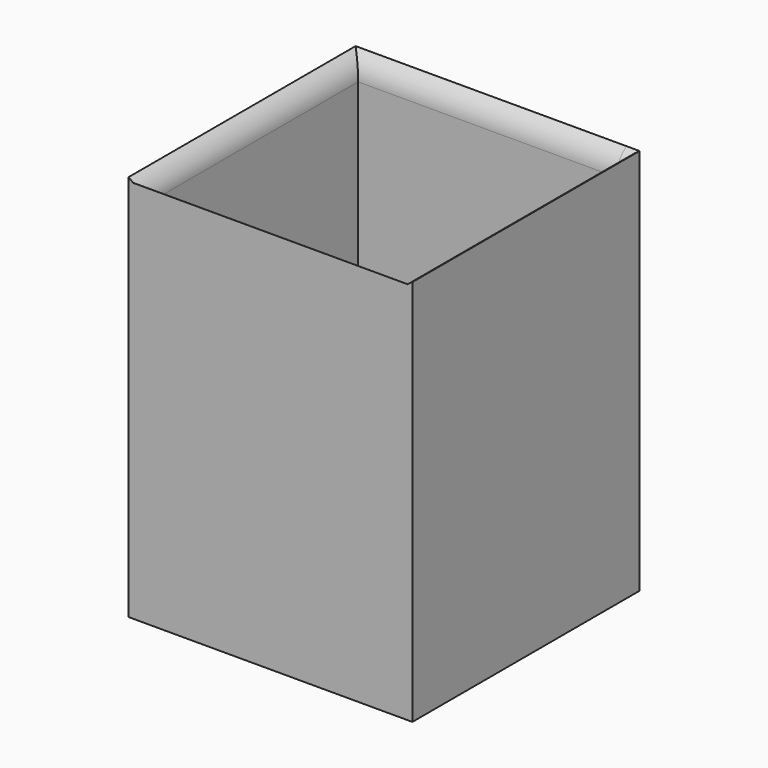
from build123d import *

# Parameters (mm, degrees)
F0_W         = 50.8
F0_H         = 50.8
F0_R         = 1.5875
F1_DEPTH     = 5.08
F0_W_2       = 55.88
F0_H_2       = 55.88
F2_DEPTH     = 76.2
F3_T1_DEPTH  = 50.8
F4_T4_DEPTH  = 64.3399164321
F4_S5_R      = 5.0800000001
F4_T6_DEPTH  = 34
F5_T4_DEPTH  = 64.3391166785
F5_S5_R      = 5.0813656856
F5_T6_DEPTH  = 34
F6_T4_DEPTH  = 77.8762455026
F6_S6_R      = 5.0800000001
F6_T7_DEPTH  = 41
F6_T11_DEPTH = 77.8762455026
F6_S13_R     = 5.081365685
F6_T14_DEPTH = 41
F7_R         = 5.7567075364
F8_DEPTH     = 8.128
F9_R         = 5.08


# Not quite as in the source:
# - a fillet or chamfer that OpenCascade refuses, or shapes differently, is made with other operations: its cross-section is extruded or revolved along the edge and cut away or added


with BuildPart() as f1:
    # F0 (on Top) → F1 (new body)
    with BuildSketch(Plane.XY):
        with Locations((0.627800245, -0.8074334759)):
            Rectangle(F0_W, F0_H)
        with Locations((-12.072199755, -13.5074334759)):
            Circle(F0_R, mode=Mode.SUBTRACT)
        with Locations((13.327800245, -13.5074334759)):
            Circle(F0_R, mode=Mode.SUBTRACT)
        with Locations((-12.072199755, 11.8925665241)):
            Circle(F0_R, mode=Mode.SUBTRACT)
        with Locations((13.327800245, 11.8925665241)):
            Circle(F0_R, mode=Mode.SUBTRACT)
    extrude(amount=F1_DEPTH)

    # F0 (on Top) → F2 (join)
    with BuildSketch(Plane.XY):
        with Locations((0.627800245, -0.8074334759)):
            Rectangle(F0_W_2, F0_H_2)
        with Locations((0.627800245, -0.8074334759)):
            Rectangle(F0_W, F0_H, mode=Mode.SUBTRACT)
    extrude(amount=F2_DEPTH)

    # F3: fillet of radius 5.08 on 1 edges, made by hand

    # F3_s2 → F3_t1 (cut)
    with BuildSketch(Plane.YZ.offset(-24.772199755)):
        with BuildLine():
            ThreePointArc((-26.2074334759, 71.12), (-27.6953310275, 74.7121024484), (-31.2874334759, 76.2))
            Line((-31.2874334759, 76.2), (-26.2074334759, 76.2))
            Line((-26.2074334759, 76.2), (-26.2074334759, 71.12))
        make_face()
    extrude(amount=F3_T1_DEPTH, mode=Mode.SUBTRACT)

    # F4: fillet of radius 5.08 on 1 edges, made by hand


with BuildPart() as f4_tool2:
    # F4_s3 → F4_t4 (new body)
    with BuildSketch(Plane.XZ.offset(-24.5925665241)):
        with BuildLine():
            ThreePointArc((-27.311999717, 76.2003463882), (-25.4524342775, 74.3404748362), (-24.771799755, 71.8000334454))
            Line((-24.771799755, 71.8000334454), (-24.2636631865, 71.8000334454))
            ThreePointArc((-24.2636631865, 71.8000334454), (-24.2640631865, 74.0000167227), (-24.2640631865, 76.2))
            Line((-24.2640631865, 76.2), (-24.772199755, 76.7081365685))
            ThreePointArc((-24.772199755, 76.7081365685), (-26.042099736, 76.7081365685), (-27.0578831447, 76.6403776825))
            Line((-27.0578831447, 76.6403776825), (-27.311999717, 76.2003463882))
        make_face()
    extrude(amount=F4_T4_DEPTH)

    # F4_s5 → F4_t6 (cut, symmetric)
    with BuildSketch(Plane.YZ.offset(-25.8)):
        with Locations((-31.287433476, 71.1199999999)):
            Circle(F4_S5_R)
    extrude(amount=F4_T6_DEPTH, both=True, mode=Mode.SUBTRACT)


with BuildPart() as f1_1:
    add(f1.part)

    # F4_t1: cut F4_tool2
    add(f4_tool2.part, mode=Mode.SUBTRACT)

    # F5: fillet of radius 5.08 on 1 edges, made by hand


with BuildPart() as f5_tool2:
    # F5_s3 → F5_t4 (new body)
    with BuildSketch(Plane.YZ.offset(26.027800245)):
        with BuildLine():
            ThreePointArc((24.5921665241, 71.8000334454), (25.2728010465, 74.3404748362), (27.1323664861, 76.2003463882))
            Line((27.1323664861, 76.2003463882), (26.8782499137, 76.6403776825))
            ThreePointArc((26.8782499137, 76.6403776825), (25.8624665051, 76.7081365685), (24.5925665241, 76.7081365685))
            Line((24.5925665241, 76.7081365685), (24.0844299555, 76.2))
            ThreePointArc((24.0844299555, 76.2), (24.0844299555, 74.0000167227), (24.0840299555, 71.8000334454))
            Line((24.0840299555, 71.8000334454), (24.5921665241, 71.8000334454))
        make_face()
    extrude(amount=-F5_T4_DEPTH)

    # F5_s5 → F5_t6 (cut, symmetric)
    with BuildSketch(Plane.XZ.offset(-25.6)):
        with Locations((-29.8531654406, 71.8000334452)):
            Circle(F5_S5_R)
    extrude(amount=F5_T6_DEPTH, both=True, mode=Mode.SUBTRACT)


with BuildPart() as f1_2:
    add(f1_1.part)

    # F5_t1: cut F5_tool2
    add(f5_tool2.part, mode=Mode.SUBTRACT)

    # F6: fillet of radius 5.08 on 1 edges, made by hand


with BuildPart() as f6_tool2:
    # F6_s3 → F6_t4 (new body)
    with BuildSketch(Plane.XZ.offset(39.745956104)):
        with BuildLine():
            ThreePointArc((28.567800245, 76.2), (26.7083911938, 74.3405909488), (26.027800245, 71.8005909488))
            Line((26.027800245, 71.8005909488), (26.027800245, 76.2))
            Line((26.027800245, 76.2), (28.567800245, 76.2))
        make_face()
    extrude(amount=-F6_T4_DEPTH)

    split(bisect_by=Plane.XZ.offset(-24.5925665241), keep=Keep.TOP)

    # F6_s6 → F6_t7 (cut, symmetric)
    with BuildSketch(Plane.YZ.offset(27.3)):
        with Locations((-31.287433476, 71.1199999999)):
            Circle(F6_S6_R)
    extrude(amount=F6_T7_DEPTH, both=True, mode=Mode.SUBTRACT)


with BuildPart() as f1_3:
    add(f1_2.part)

    # F6_t1: cut F6_tool2
    add(f6_tool2.part, mode=Mode.SUBTRACT)


with BuildPart() as f6_tool9:
    # F6_s10 → F6_t11 (new body)
    with BuildSketch(Plane.XZ.offset(39.745956104)):
        with BuildLine():
            ThreePointArc((28.567800245, 76.2), (26.7083911938, 74.3405909488), (26.027800245, 71.8005909488))
            Line((26.027800245, 71.8005909488), (26.027800245, 76.2))
            Line((26.027800245, 76.2), (28.567800245, 76.2))
        make_face()
    extrude(amount=-F6_T11_DEPTH)

    split(bisect_by=Plane.XZ.offset(-24.5925665241), keep=Keep.BOTTOM)

    # F6_s13 → F6_t14 (cut, symmetric)
    with BuildSketch(Plane.YZ.offset(27.3)):
        with Locations((29.6735322091, 71.8000334456)):
            Circle(F6_S13_R)
    extrude(amount=F6_T14_DEPTH, both=True, mode=Mode.SUBTRACT)


with BuildPart() as f1_4:
    add(f1_3.part)

    # F6_t8: cut F6_tool9
    add(f6_tool9.part, mode=Mode.SUBTRACT)

    # F7 (on face) → F8 (join)
    with BuildSketch(Plane(origin=(0, 27.1325665241, 0), x_dir=(-1, 0, 0), z_dir=(0, 1, 0))):
        with Locations((0, 38.1)):
            Circle(F7_R)
    extrude(amount=F8_DEPTH)

    # F9
    f9_edges = [f1_4.edges().sort_by_distance(p)[0] for p in [
        (5.756708, 35.260567, 38.1),
    ]]
    fillet(f9_edges, radius=F9_R)


solid = f1_4.part
